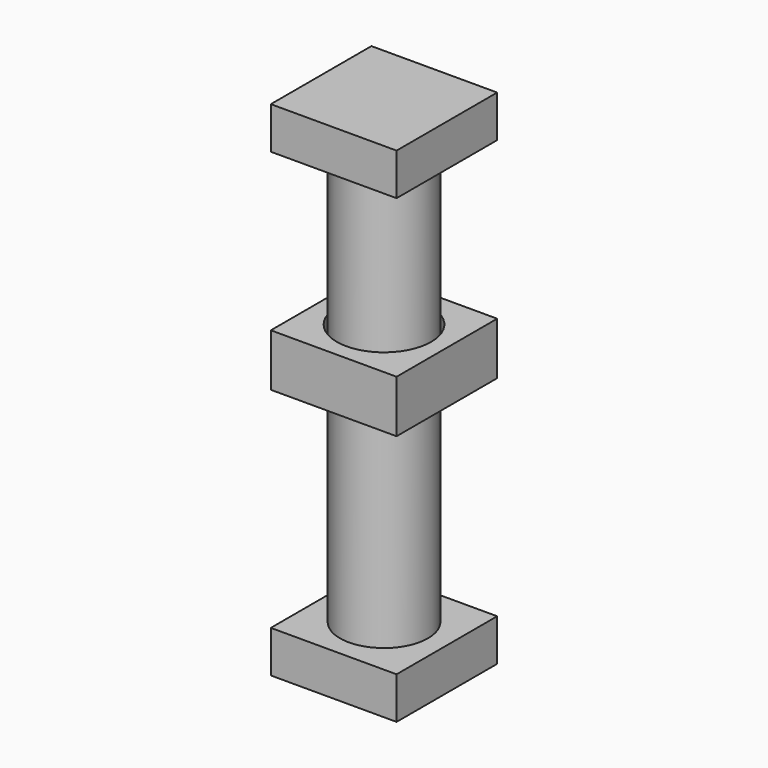
from build123d import *

# Parameters (mm, degrees)
F0_W     = 60
F0_H     = 60
F1_DEPTH = 25
F2_R     = 22.5
F3_DEPTH = 25.001
F4_R     = 21
F5_DEPTH = 100
F6_W     = 60
F6_H     = 60
F6_R     = 21
F7_DEPTH = 20
F8_W     = 60
F8_H     = 60
F8_R     = 21
F9_DEPTH = 20


with BuildPart() as f1:
    # F0 (on Top) → F1 (new body)
    with BuildSketch(Plane.XY):
        Rectangle(F0_W, F0_H)
    extrude(amount=F1_DEPTH)

    # F2 (on face) → F3 (cut, through all)
    with BuildSketch(Plane.XY.offset(25)):
        Circle(F2_R)
    extrude(amount=-F3_DEPTH, mode=Mode.SUBTRACT)


with BuildPart() as f5:
    # F4 (on Top) → F5 (new body, symmetric)
    with BuildSketch(Plane.XY):
        Circle(F4_R)
    extrude(amount=F5_DEPTH, both=True)

    # F6 (on face) → F7 (join)
    with BuildSketch(Plane.XY.offset(100)):
        Rectangle(F6_W, F6_H)
        Circle(F6_R, mode=Mode.SUBTRACT)
        Circle(F6_R)
    extrude(amount=F7_DEPTH)

    # F8 (on face) → F9 (join)
    with BuildSketch(Plane(origin=(0, 0, -100), x_dir=(1, 0, 0), z_dir=(0, 0, -1))):
        Rectangle(F8_W, F8_H)
        Circle(F8_R, mode=Mode.SUBTRACT)
        Circle(F8_R)
    extrude(amount=F9_DEPTH)


solid = Compound([f1.part, f5.part])
